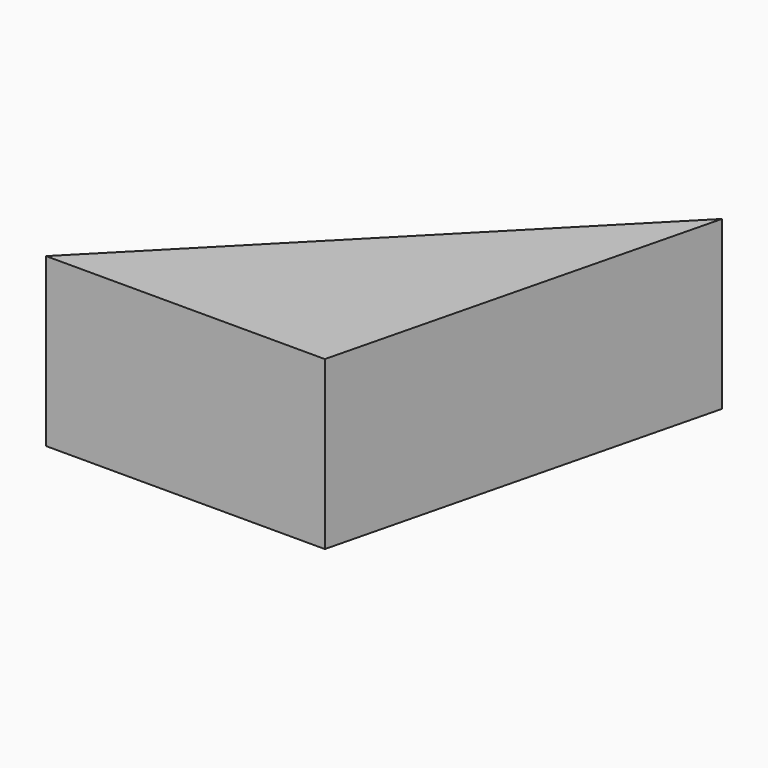
from build123d import *

# Parameters (mm, degrees)
F1_DEPTH = 76.2
F3_DEPTH = 2


# Not quite as in the source:
# - a feature of the source that left no trace in its solid (it failed there, or was rolled back) is left out


with BuildPart() as f1:
    # F0 (on Top) → F1 (new body)
    with BuildSketch(Plane.XY):
        Polygon((-103.2740693459, -42.971104271), (23.7259306541, -42.971104271), (66.5791147949, 129.5874208994), align=None)
    extrude(amount=F1_DEPTH)

    # F2 (on face) → F3 (join)
    with BuildSketch(Plane(origin=(0, 0, 0), x_dir=(1, 0, 0), z_dir=(0, 0, -1))):
        Polygon((23.7259306541, 42.971104271), (-103.2740693459, 42.971104271), (66.5791147949, -129.5874208994), align=None)
    extrude(amount=-F3_DEPTH)


solid = f1.part
